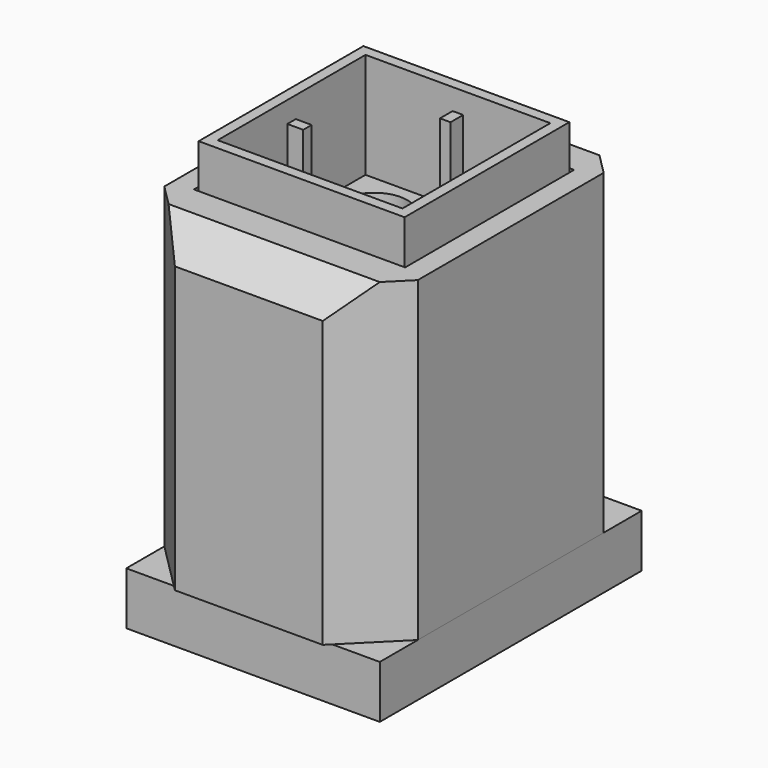
from build123d import *

# Parameters (mm, degrees)
F0_W          = 19.5
F0_H          = 19.5
F1_DEPTH      = 13
F2_W          = 19.5
F2_H          = 19.5
F2_W_2        = 17.5
F2_H_2        = 17.5
F3_DEPTH      = 10
F4_W          = 1
F4_H          = 1.5
F4_W_2        = 1.5
F4_H_2        = 1
F5_DEPTH      = 8
F6_R          = 3.1
F7_DEPTH      = 19
F8_W          = 1
F8_H          = 19.5
F9_DEPTH      = 9
F10_R         = 2.55
F11_DEPTH     = 3
F13_W         = 20
F13_H         = 20
F13_W_2       = 10
F13_H_2       = 5
F14_DEPTH     = 30
F15_W         = 22
F15_H         = 20
F16_DEPTH     = 20
F17_R         = 1.2
F18_DEPTH     = 6
F19_T4_DEPTH  = 30
F19_T10_DEPTH = 30
F19_T16_DEPTH = 30
F19_T22_DEPTH = 30
F20_R         = 1.2
F21_DEPTH     = 10
F23_W         = 24
F23_H         = 31
F23_R         = 1.5
F23_R_2       = 2.75
F23_R_3       = 4
F24_DEPTH     = 5
F25_SIZE      = 3


# Not quite as in the source:
# - a fillet or chamfer that OpenCascade refuses, or shapes differently, is made with other operations: its cross-section is extruded or revolved along the edge and cut away or added


with BuildPart() as f1:
    # F0 (on Top) → F1 (new body)
    with BuildSketch(Plane.XY):
        Rectangle(F0_W, F0_H)
    extrude(amount=F1_DEPTH)

    # F2 (on face) → F3 (join)
    with BuildSketch(Plane.XY.offset(13)):
        Rectangle(F2_W, F2_H)
        Rectangle(F2_W_2, F2_H_2, mode=Mode.SUBTRACT)
    extrude(amount=F3_DEPTH)

    # F4 (on face) → F5 (join)
    with BuildSketch(Plane.XY.offset(13)):
        with Locations((0, 8)):
            Rectangle(F4_W, F4_H)
        with Locations((0, -8)):
            Rectangle(F4_W, F4_H)
        with Locations((-8, 0)):
            Rectangle(F4_W_2, F4_H_2)
        with Locations((8, 0)):
            Rectangle(F4_W_2, F4_H_2)
    extrude(amount=F5_DEPTH)

    # F6 (on face) → F7 (cut)
    with BuildSketch(Plane.XY.offset(13)):
        with Locations((-4.5, 4.5)):
            Circle(F6_R)
        with Locations((-4.5, -4.5)):
            Circle(F6_R)
        with Locations((4.5, 4.5)):
            Circle(F6_R)
        with Locations((4.5, -4.5)):
            Circle(F6_R)
    extrude(amount=-F7_DEPTH, mode=Mode.SUBTRACT)

    # F8 (on face) → F9 (join)
    with BuildSketch(Plane(origin=(0, 0, 0), x_dir=(1, 0, 0), z_dir=(0, 0, -1))):
        with Locations((-10.25, 0)):
            Rectangle(F8_W, F8_H)
        with Locations((10.25, 0)):
            Rectangle(F8_W, F8_H)
    extrude(amount=-F9_DEPTH)

    # F10 (on face) → F11 (cut)
    with BuildSketch(Plane(origin=(0, 0, 0), x_dir=(1, 0, 0), z_dir=(0, 0, -1))):
        Circle(F10_R)
    extrude(amount=-F11_DEPTH, mode=Mode.SUBTRACT)


with BuildPart() as f14:
    # F13 (on offset) → F14 (new body)
    with BuildSketch(Plane.XY.offset(19)):
        Polygon((5, -11), (12, -11), (12, 11), (5, 11), (-5, 11), (-12, 11), (-12, -11), (-5, -11), align=None)
        Rectangle(F13_W, F13_H, mode=Mode.SUBTRACT)
        with Locations((0, -13.5)):
            Rectangle(F13_W_2, F13_H_2)
        with Locations((0, 13.5)):
            Rectangle(F13_W_2, F13_H_2)
    extrude(amount=-F14_DEPTH)

    # F15 (on face) → F16 (cut)
    with BuildSketch(Plane(origin=(0, 0, -11), x_dir=(1, 0, 0), z_dir=(0, 0, -1))):
        Rectangle(F15_W, F15_H)
    extrude(amount=-F16_DEPTH, mode=Mode.SUBTRACT)

    # F17 (on face) → F18 (cut)
    with BuildSketch(Plane(origin=(0, 16, 0), x_dir=(-1, 0, 0), z_dir=(0, 1, 0))):
        with Locations((0, 10.5)):
            Circle(F17_R)
        with Locations((0, -4.5)):
            Circle(F17_R)
    extrude(amount=-F18_DEPTH, mode=Mode.SUBTRACT)

    # F19: chamfer of 7 on 4 edges, made by hand


with BuildPart() as f19_tool2:
    # F19_s3 → F19_t4 (new body)
    with BuildSketch(Plane.XY.offset(19)):
        Polygon((12, 11), (5, 18), (5, 11), align=None)
    extrude(amount=-F19_T4_DEPTH)

    split(bisect_by=Plane.YZ.offset(12), keep=Keep.BOTTOM)

    split(bisect_by=Plane.XZ.offset(-16), keep=Keep.TOP)


with BuildPart() as f14_1:
    add(f14.part)

    # F19_t1: union F19_tool2
    add(f19_tool2.part)


with BuildPart() as f19_tool8:
    # F19_s9 → F19_t10 (new body)
    with BuildSketch(Plane.XY.offset(19)):
        Polygon((-5, 18), (-12, 11), (-5, 11), align=None)
    extrude(amount=-F19_T10_DEPTH)

    split(bisect_by=Plane.XZ.offset(-16), keep=Keep.TOP)

    split(bisect_by=Plane.YZ.offset(-12), keep=Keep.TOP)


with BuildPart() as f14_2:
    add(f14_1.part)

    # F19_t7: union F19_tool8
    add(f19_tool8.part)


with BuildPart() as f19_tool14:
    # F19_s15 → F19_t16 (new body)
    with BuildSketch(Plane.XY.offset(19)):
        Polygon((-12, -11), (-5, -18), (-5, -11), align=None)
    extrude(amount=-F19_T16_DEPTH)

    split(bisect_by=Plane.XZ.offset(16), keep=Keep.BOTTOM)

    split(bisect_by=Plane.YZ.offset(-12), keep=Keep.TOP)


with BuildPart() as f14_3:
    add(f14_2.part)

    # F19_t13: union F19_tool14
    add(f19_tool14.part)


with BuildPart() as f19_tool20:
    # F19_s21 → F19_t22 (new body)
    with BuildSketch(Plane.XY.offset(19)):
        Polygon((12, -11), (5, -18), (5, -11), align=None)
    extrude(amount=-F19_T22_DEPTH)

    split(bisect_by=Plane.YZ.offset(12), keep=Keep.BOTTOM)

    split(bisect_by=Plane.XZ.offset(16), keep=Keep.BOTTOM)


with BuildPart() as f14_4:
    add(f14_3.part)

    # F19_t19: union F19_tool20
    add(f19_tool20.part)

    # F20 (on face) → F21 (cut)
    with BuildSketch(Plane(origin=(0, 0, -11), x_dir=(1, 0, 0), z_dir=(0, 0, -1))):
        with Locations((0, 13)):
            Circle(F20_R)
        with Locations((-5, -13)):
            Circle(F20_R)
        with Locations((5, -13)):
            Circle(F20_R)
    extrude(amount=-F21_DEPTH, mode=Mode.SUBTRACT)

    # F25
    f25_edges = [f14_4.edges().sort_by_distance(p)[0] for p in [
        (0, 16, 19),
        (0, -16, 19),
    ]]
    chamfer(f25_edges, length=F25_SIZE)


with BuildPart() as f24:
    # F23 (on offset) → F24 (new body)
    with BuildSketch(Plane(origin=(0, 0, -11), x_dir=(1, 0, 0), z_dir=(0, 0, -1))):
        Rectangle(F23_W, F23_H)
        with Locations((-5, -13)):
            Circle(F23_R, mode=Mode.SUBTRACT)
        with Locations((-5.5, -5.5)):
            Circle(F23_R_2, mode=Mode.SUBTRACT)
        with Locations((5, -13)):
            Circle(F23_R, mode=Mode.SUBTRACT)
        with Locations((5.5, -5.5)):
            Circle(F23_R_2, mode=Mode.SUBTRACT)
        with Locations((-5.5, 5.5)):
            Circle(F23_R_2, mode=Mode.SUBTRACT)
        Circle(F23_R_3, mode=Mode.SUBTRACT)
        with Locations((5.5, 5.5)):
            Circle(F23_R_2, mode=Mode.SUBTRACT)
        with Locations((0, 13)):
            Circle(F23_R, mode=Mode.SUBTRACT)
    extrude(amount=F24_DEPTH)


solid = Compound([f1.part, f14_4.part, f24.part])
